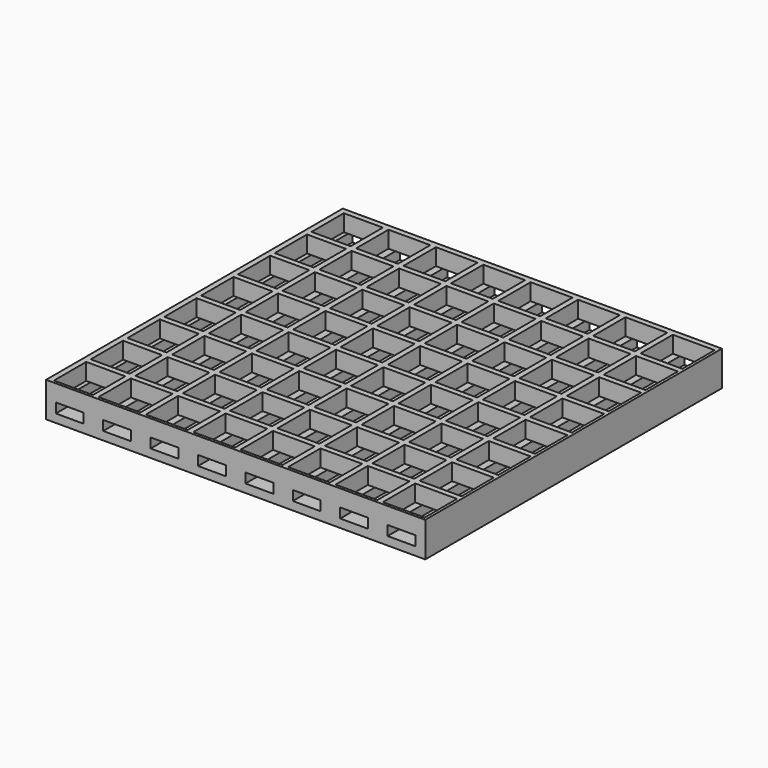
from build123d import *

# Parameters (mm, degrees)
F0_W                 = 3.5
F0_H                 = 3.5
F0_W_2               = 7
F1_DEPTH             = 133
F2_W                 = 2
F2_H                 = 6
F2_W_2               = 1
F3_DEPTH             = 133
F4_W                 = 2
F4_H                 = 6
F4_W_2               = 1
F5_DEPTH             = 136
F8_D                 = 3.5
F8_DEPTH             = 12
F8_CSINK_D           = 6.5
F8_CSINK_ANGLE       = 90
F8_TIP               = 1.0515060833
F8_ON_F6_D           = 3.5
F8_ON_F6_DEPTH       = 12
F8_ON_F6_CSINK_D     = 6.5
F8_ON_F6_CSINK_ANGLE = 90
F8_ON_F6_TIP         = 1.0515060833


# Not quite as in the source:
# - a feature names something its author has since deleted; it is built from what else it names


with BuildPart() as f1:
    # F0 (on Front) → F1 (new body)
    with BuildSketch(Plane.XZ):
        with Locations((-66.25, 4.75)):
            Rectangle(F0_W, F0_H)
        with Locations((-17, 4.75)):
            Rectangle(F0_W_2, F0_H)
        with Locations((66.25, 4.75)):
            Rectangle(F0_W, F0_H)
        Polygon((-64.5, 3), (-68, 3), (-68, 0), (68, 0), (68, 3), (64.5, 3), (54.5, 3), (47.5, 3), (37.5, 3), (30.5, 3), (20.5, 3), (13.5, 3), (3.5, 3), (-3.5, 3), (-13.5, 3), (-20.5, 3), (-30.5, 3), (-37.5, 3), (-47.5, 3), (-54.5, 3), align=None)
        with Locations((-51, 4.75)):
            Rectangle(F0_W_2, F0_H)
        with Locations((-34, 4.75)):
            Rectangle(F0_W_2, F0_H)
        with Locations((0, 4.75)):
            Rectangle(F0_W_2, F0_H)
        with Locations((17, 4.75)):
            Rectangle(F0_W_2, F0_H)
        with Locations((34, 4.75)):
            Rectangle(F0_W_2, F0_H)
        with Locations((51, 4.75)):
            Rectangle(F0_W_2, F0_H)
    extrude(amount=F1_DEPTH)

    # F2 (on face) → F3 (join, through all)
    with BuildSketch(Plane.XZ.offset(133)):
        with Locations((-67, 9.5)):
            Rectangle(F2_W, F2_H)
        with Locations((-51, 9.5)):
            Rectangle(F2_W, F2_H)
        with Locations((-34, 9.5)):
            Rectangle(F2_W, F2_H)
        with Locations((-17, 9.5)):
            Rectangle(F2_W, F2_H)
        with Locations((0, 9.5)):
            Rectangle(F2_W, F2_H)
        with Locations((17, 9.5)):
            Rectangle(F2_W, F2_H)
        with Locations((34, 9.5)):
            Rectangle(F2_W, F2_H)
        with Locations((51, 9.5)):
            Rectangle(F2_W, F2_H)
        with Locations((67.5, 9.5)):
            Rectangle(F2_W_2, F2_H)
    extrude(amount=-F3_DEPTH)

    # F4 (on face) → F5 (join, through all)
    with BuildSketch(Plane(origin=(-68, 0, 0), x_dir=(0, -1, 0), z_dir=(-1, 0, 0))):
        with Locations((1, 9.5)):
            Rectangle(F4_W, F4_H)
        with Locations((17.5, 9.5)):
            Rectangle(F4_W, F4_H)
        with Locations((34, 9.5)):
            Rectangle(F4_W, F4_H)
        with Locations((50.5, 9.5)):
            Rectangle(F4_W, F4_H)
        with Locations((67, 9.5)):
            Rectangle(F4_W, F4_H)
        with Locations((83.5, 9.5)):
            Rectangle(F4_W, F4_H)
        with Locations((100, 9.5)):
            Rectangle(F4_W, F4_H)
        with Locations((116.5, 9.5)):
            Rectangle(F4_W, F4_H)
        with Locations((132.5, 9.5)):
            Rectangle(F4_W_2, F4_H)
    extrude(amount=-F5_DEPTH)

    # F8
    with Locations(Plane.XY.offset(3)):
        with Locations((42.5, -42), (42.5, -91)):
            CounterSinkHole(F8_D / 2, F8_CSINK_D / 2, depth=F8_DEPTH, counter_sink_angle=F8_CSINK_ANGLE)
            with Locations((0, 0, -(F8_DEPTH + F8_TIP / 2))):  # 118° drill point
                Cone(0, F8_D / 2, F8_TIP, mode=Mode.SUBTRACT)

    # F8 on F6
    with Locations(Plane.XY.offset(3)):
        with Locations((-42.5, -42), (-42.5, -91)):
            CounterSinkHole(F8_ON_F6_D / 2, F8_ON_F6_CSINK_D / 2, depth=F8_ON_F6_DEPTH, counter_sink_angle=F8_ON_F6_CSINK_ANGLE)
            with Locations((0, 0, -(F8_ON_F6_DEPTH + F8_ON_F6_TIP / 2))):  # 118° drill point
                Cone(0, F8_ON_F6_D / 2, F8_ON_F6_TIP, mode=Mode.SUBTRACT)


solid = f1.part
